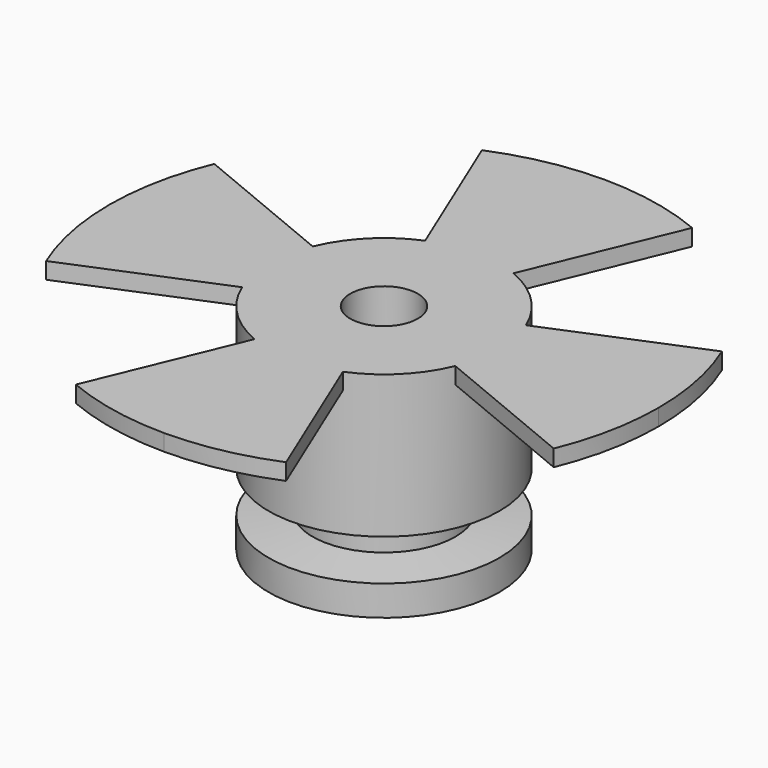
from build123d import *

# Parameters (mm, degrees)
F0_R      = 10.5
F0_R_2    = 6.5
F0_R_3    = 3.075
F1_DEPTH  = 3.25
F2_DEPTH  = 6
F3_R      = 10.5
F3_R_2    = 6.5
F3_R_3    = 3.075
F4_DEPTH  = 12
F6_DEPTH  = 1.5
F7_DEPTH  = 1.5
F8_R      = 1.55
F9_DEPTH  = 20
F10_SIZE2 = 0.5
F10_SIZE  = 5
F11_SIZE2 = 5
F11_SIZE  = 0.5
F12_DEPTH = 1


with BuildPart() as f1:
    # F0 (on Top) → F1 (new body)
    with BuildSketch(Plane.XY):
        Circle(F0_R)
        Circle(F0_R_2, mode=Mode.SUBTRACT)
        Circle(F0_R_2)
        Circle(F0_R_3, mode=Mode.SUBTRACT)
    extrude(amount=F1_DEPTH)

    # F10
    f10_edges = [f1.edges().sort_by_distance(p)[0] for p in [
        (-10.5, 0, 3.25),
    ]]
    f10_side = f1.faces().sort_by_distance((-3.371985, 0, 3.25))[0]
    chamfer(f10_edges, length=F10_SIZE, length2=F10_SIZE2, reference=f10_side)


with BuildPart() as f2:
    # F0 (on Top) → F2 (new body)
    with BuildSketch(Plane.XY):
        Circle(F0_R_2)
        Circle(F0_R_3, mode=Mode.SUBTRACT)
    extrude(amount=F2_DEPTH)

    # F12 (add): a face of the model
    f12_faces = [f2.faces().sort_by_distance(p)[0] for p in [
        (-6.3161522369, 0, 6),
    ]]
    extrude(f12_faces, amount=F12_DEPTH)


with BuildPart() as f4:
    # F3 (on face) → F4 (new body)
    with BuildSketch(Plane.XY.offset(6)):
        Circle(F3_R)
        Circle(F3_R_2, mode=Mode.SUBTRACT)
        Circle(F3_R_2)
        Circle(F3_R_3, mode=Mode.SUBTRACT)
    extrude(amount=F4_DEPTH)

    # F5 (on face) → F6 (join)
    with BuildSketch(Plane.XY.offset(18)):
        with BuildLine():
            Line((-25, 0), (-10.5, 0))
            ThreePointArc((-10.5, 0), (-10.2982454442, 2.0484483812), (-9.7007350914, 4.0181760398))
            Line((-9.7007350914, 4.0181760398), (-23.0969883128, 9.5670858091))
            ThreePointArc((-23.0969883128, 9.5670858091), (-24.5196320101, 4.8772580504), (-25, 0))
        make_face()
        with BuildLine():
            ThreePointArc((-9.7007350914, -4.0181760398), (-10.2982454442, -2.0484483812), (-10.5, 0))
            Line((-10.5, 0), (-25, 0))
            ThreePointArc((-25, 0), (-24.5196320101, -4.8772580504), (-23.0969883128, -9.5670858091))
            Line((-23.0969883128, -9.5670858091), (-9.7007350914, -4.0181760398))
        make_face()
        with BuildLine():
            ThreePointArc((-9.5670858091, -23.0969883128), (-4.8772580504, -24.5196320101), (0, -25))
            Line((0, -25), (0, -10.5))
            ThreePointArc((0, -10.5), (-2.0484483812, -10.2982454442), (-4.0181760398, -9.7007350914))
            Line((-4.0181760398, -9.7007350914), (-9.5670858091, -23.0969883128))
        make_face()
        with BuildLine():
            ThreePointArc((0, -25), (4.8772580504, -24.5196320101), (9.5670858091, -23.0969883128))
            Line((9.5670858091, -23.0969883128), (4.0181760398, -9.7007350914))
            ThreePointArc((4.0181760398, -9.7007350914), (2.0484483812, -10.2982454442), (0, -10.5))
            Line((0, -10.5), (0, -25))
        make_face()
        with BuildLine():
            ThreePointArc((23.0969883128, -9.5670858091), (24.5196320101, -4.8772580504), (25, 0))
            Line((25, 0), (10.5, 0))
            ThreePointArc((10.5, 0), (10.2982454442, -2.0484483812), (9.7007350914, -4.0181760398))
            Line((9.7007350914, -4.0181760398), (23.0969883128, -9.5670858091))
        make_face()
        with BuildLine():
            Line((10.5, 0), (25, 0))
            ThreePointArc((25, 0), (24.5196320101, 4.8772580504), (23.0969883128, 9.5670858091))
            Line((23.0969883128, 9.5670858091), (9.7007350914, 4.0181760398))
            ThreePointArc((9.7007350914, 4.0181760398), (10.2982454442, 2.0484483812), (10.5, 0))
        make_face()
        with BuildLine():
            Line((4.0181760398, 9.7007350914), (9.5670858091, 23.0969883128))
            ThreePointArc((9.5670858091, 23.0969883128), (4.8772580504, 24.5196320101), (0, 25))
            Line((0, 25), (0, 10.5))
            ThreePointArc((0, 10.5), (2.0484483812, 10.2982454442), (4.0181760398, 9.7007350914))
        make_face()
        with BuildLine():
            Line((0, 10.5), (0, 25))
            ThreePointArc((0, 25), (-4.8772580504, 24.5196320101), (-9.5670858091, 23.0969883128))
            Line((-9.5670858091, 23.0969883128), (-4.0181760398, 9.7007350914))
            ThreePointArc((-4.0181760398, 9.7007350914), (-2.0484483812, 10.2982454442), (0, 10.5))
        make_face()
    extrude(amount=F6_DEPTH)

    # F7 (add): a face of the model
    f7_faces = [f4.faces().sort_by_distance(p)[0] for p in [
        (10.0069670767, 1.9905095115, 18),
    ]]
    extrude(f7_faces, amount=F7_DEPTH)

    # F8 (on Front) → F9 (cut)
    with BuildSketch(Plane.XZ):
        with Locations((0, 9.9058225751)):
            Circle(F8_R)
    extrude(amount=-F9_DEPTH, mode=Mode.SUBTRACT)

    # F11
    f11_edges = [f4.edges().sort_by_distance(p)[0] for p in [
        (-10.5, 0, 6),
    ]]
    f11_side = f4.faces().sort_by_distance((-10.5, 0, 12.75))[0]
    chamfer(f11_edges, length=F11_SIZE, length2=F11_SIZE2, reference=f11_side)


solid = Compound([f1.part, f2.part, f4.part])
